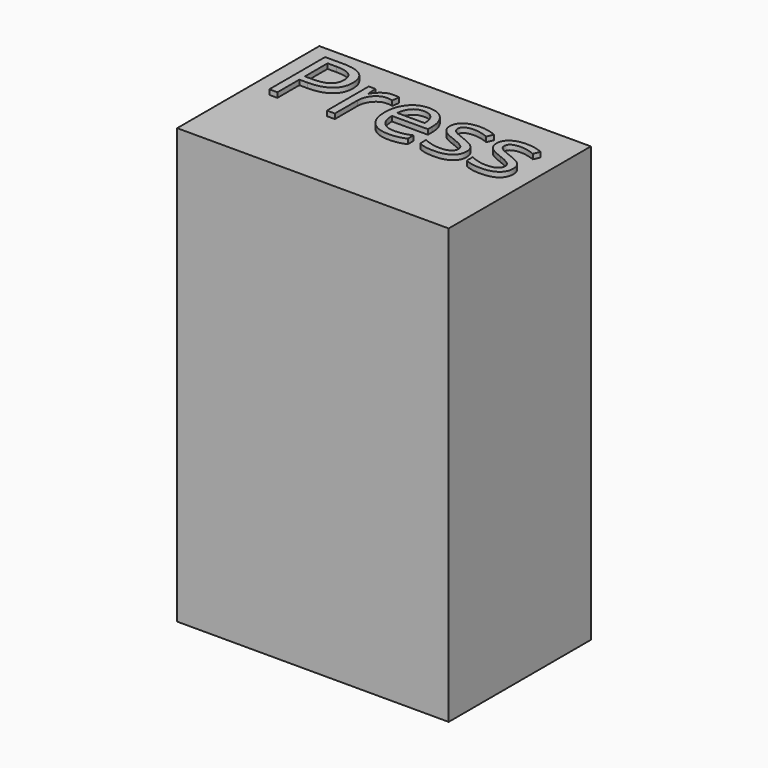
from build123d import *

# Parameters (mm, degrees)
F0_W         = 1397
F0_H         = 914.4
F1_DEPTH     = 2235.2
F2_TEXT_SIZE = 502.7083473073
F3_DEPTH     = 25.4


# Not quite as in the source:
# - Text() gives the source's letters only with a copy of the font that has no kerning and outlines rounded to 1/6400 em; it was checked with that copy


with BuildPart() as f1:
    # F0 (on Top) → F1 (new body)
    with BuildSketch(Plane.XY):
        Rectangle(F0_W, F0_H)
    extrude(amount=F1_DEPTH)

    # F2 (on face) → F3 (join)
    with BuildSketch(Plane.XY.offset(2235.2)):
        with Locations((-639.53927559, 0)):
            Text('Press', F2_TEXT_SIZE, font='Open Sans', text_align=(TextAlign.LEFT, TextAlign.BOTTOM))
    extrude(amount=F3_DEPTH)


solid = f1.part
